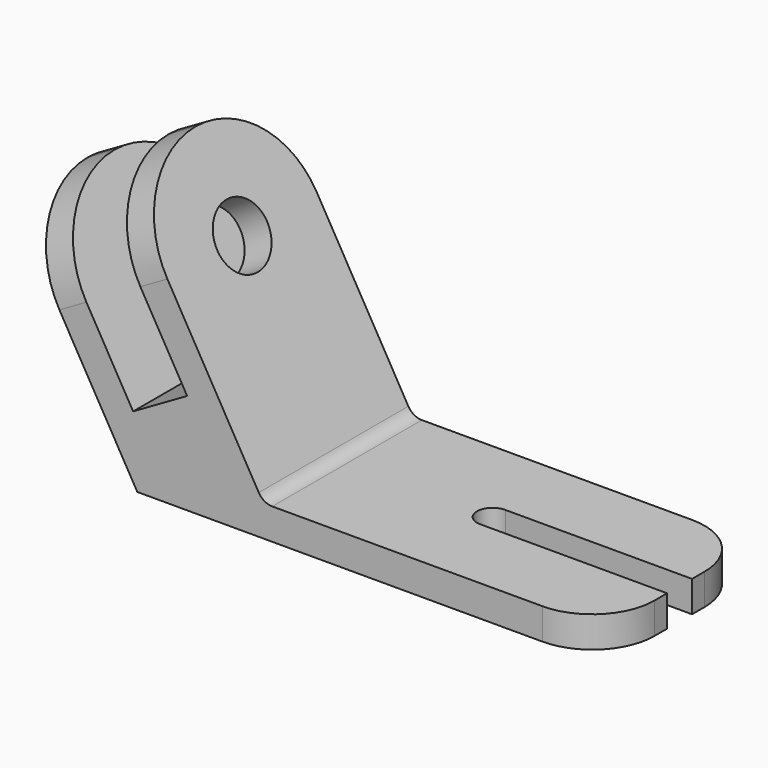
from build123d import *

# Parameters (mm, degrees)
F1_DEPTH = 60
F2_R     = 20
F4_DEPTH = 10.001
F5_R     = 29.99999
F7_D     = 20


# Not quite as in the source:
# - a fillet or chamfer is up to 0.001 mm smaller than in the source, because OpenCascade refuses the exact size


with BuildPart() as f1:
    # F0 (on Front) → F1 (new body)
    with BuildSketch(Plane.XZ):
        with BuildLine():
            Line((-40, 69.2820323028), (0, 0))
            Line((0, 0), (150, 0))
            Line((150, 0), (150, 10))
            Line((150, 10), (43.3012701892, 10))
            ThreePointArc((43.3012701892, 10), (40.8012701892, 10.6698729811), (38.9711431703, 12.5))
            Line((38.9711431703, 12.5), (-5.3589838486, 89.2820323028))
            Line((-5.3589838486, 89.2820323028), (-14.0192378865, 84.2820323028))
            Line((-14.0192378865, 84.2820323028), (15.9807621135, 32.3205080757))
            Line((15.9807621135, 32.3205080757), (-1.3397459622, 22.3205080757))
            Line((-1.3397459622, 22.3205080757), (-31.3397459622, 74.2820323028))
            Line((-31.3397459622, 74.2820323028), (-40, 69.2820323028))
        make_face()
    extrude(amount=F1_DEPTH)

    # F2
    f2_edges = [f1.edges().sort_by_distance(p)[0] for p in [
        (150, 0, 5),
        (150, -60, 5),
    ]]
    fillet(f2_edges, radius=F2_R)

    # F3 (on face) → F4 (cut, through all)
    with BuildSketch(Plane.XY.offset(10)):
        with BuildLine():
            ThreePointArc((90, -35), (93.5355339059, -33.5355339059), (95, -30))
            ThreePointArc((95, -30), (93.5818777161, -26.5114255022), (90.1319391892, -25.0017410981))
            ThreePointArc((90.1319391892, -25.0017410981), (85.0004352935, -29.9340246617), (90, -35))
        make_face()
        with BuildLine():
            ThreePointArc((90.1319391892, -25.0017410981), (93.5818777161, -26.5114255022), (95, -30))
            ThreePointArc((95, -30), (93.5355339059, -33.5355339059), (90, -35))
            Line((90, -35), (150, -35))
            Line((150, -35), (150, -25.0017410981))
            Line((150, -25.0017410981), (90.1319391892, -25.0017410981))
        make_face()
    extrude(amount=-F4_DEPTH, mode=Mode.SUBTRACT)

    # F5 (radius 30 in the source; OpenCascade refuses exactly that, so slightly less here)
    f5_edges = [f1.edges().sort_by_distance(p)[0] for p in [
        (-9.689111, -60, 86.782032),
        (-9.689111, 0, 86.782032),
        (-35.669873, -60, 71.782032),
        (-35.669873, 0, 71.782032),
    ]]
    fillet(f5_edges, radius=F5_R)

    # F7 (through all)
    with Locations(Plane(origin=(34.6410161514, 0, 20), x_dir=(0, 1, 0), z_dir=(0.8660254038, 0, 0.5))):
        with Locations((-30, 50)):
            Hole(F7_D / 2)


solid = f1.part
